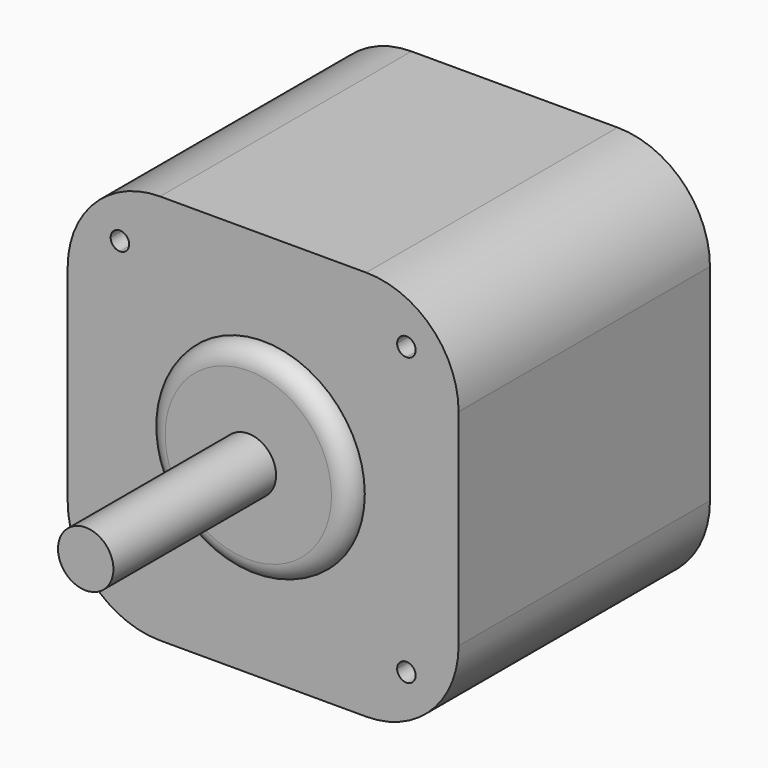
from build123d import *

# Parameters (mm, degrees)
F0_W     = 42.3
F0_H     = 42.3
F1_DEPTH = 34
F2_R     = 3
F3_DEPTH = 24
F5_DEPTH = 58.001
F6_R     = 11
F7_DEPTH = 2
F8_R     = 10
F9_R     = 1.99999


# Not quite as in the source:
# - a fillet or chamfer is up to 0.001 mm smaller than in the source, because OpenCascade refuses the exact size


with BuildPart() as f1:
    # F0 (on Front) → F1 (new body)
    with BuildSketch(Plane.XZ):
        Rectangle(F0_W, F0_H)
    extrude(amount=F1_DEPTH)

    # F2 (on face) → F3 (join)
    with BuildSketch(Plane.XZ.offset(34)):
        Circle(F2_R)
    extrude(amount=F3_DEPTH)

    # F4 (on face) → F5 (cut, through all)
    with BuildSketch(Plane(origin=(0, 0, 0), x_dir=(-1, 0, 0), z_dir=(0, 1, 0))):
        with BuildLine():
            Line((-15.5, 14.5), (-15.5, 15.5))
            Line((-15.5, 15.5), (-14.5, 15.5))
            ThreePointArc((-14.5, 15.5), (-16.2071067812, 16.2071067812), (-15.5, 14.5))
        make_face()
        with BuildLine():
            ThreePointArc((16.5, 15.5), (15.5, 16.5), (14.5, 15.5))
            Line((14.5, 15.5), (15.5, 15.5))
            Line((15.5, 15.5), (15.5, 14.5))
            ThreePointArc((15.5, 14.5), (16.2071067812, 14.7928932188), (16.5, 15.5))
        make_face()
        with BuildLine():
            Line((-15.5, -15.5), (-15.5, -14.5))
            ThreePointArc((-15.5, -14.5), (-16.2071067812, -16.2071067812), (-14.5, -15.5))
            Line((-14.5, -15.5), (-15.5, -15.5))
        make_face()
        with BuildLine():
            ThreePointArc((16.5, -15.5), (16.2071067812, -14.7928932188), (15.5, -14.5))
            Line((15.5, -14.5), (15.5, -15.5))
            Line((15.5, -15.5), (14.5, -15.5))
            ThreePointArc((14.5, -15.5), (15.5, -16.5), (16.5, -15.5))
        make_face()
        with BuildLine():
            Line((15.5, 15.5), (14.5, 15.5))
            ThreePointArc((14.5, 15.5), (14.7928932188, 14.7928932188), (15.5, 14.5))
            Line((15.5, 14.5), (15.5, 15.5))
        make_face()
        with BuildLine():
            Line((-14.5, 15.5), (-15.5, 15.5))
            Line((-15.5, 15.5), (-15.5, 14.5))
            ThreePointArc((-15.5, 14.5), (-14.7928932188, 14.7928932188), (-14.5, 15.5))
        make_face()
        with BuildLine():
            ThreePointArc((-14.5, -15.5), (-14.7928932188, -14.7928932188), (-15.5, -14.5))
            Line((-15.5, -14.5), (-15.5, -15.5))
            Line((-15.5, -15.5), (-14.5, -15.5))
        make_face()
        with BuildLine():
            Line((15.5, -15.5), (15.5, -14.5))
            ThreePointArc((15.5, -14.5), (14.7928932188, -14.7928932188), (14.5, -15.5))
            Line((14.5, -15.5), (15.5, -15.5))
        make_face()
    extrude(amount=-F5_DEPTH, mode=Mode.SUBTRACT)

    # F6 (on face) → F7 (join)
    with BuildSketch(Plane.XZ.offset(34)):
        Circle(F6_R)
    extrude(amount=F7_DEPTH)

    # F8
    f8_edges = [f1.edges().sort_by_distance(p)[0] for p in [
        (21.15, -17, 21.15),
        (-21.15, -17, 21.15),
        (21.15, -17, -21.15),
        (-21.15, -17, -21.15),
    ]]
    fillet(f8_edges, radius=F8_R)

    # F9 (radius 2 in the source; OpenCascade refuses exactly that, so slightly less here)
    f9_edges = [f1.edges().sort_by_distance(p)[0] for p in [
        (-11, -36, 0),
    ]]
    fillet(f9_edges, radius=F9_R)


solid = f1.part
